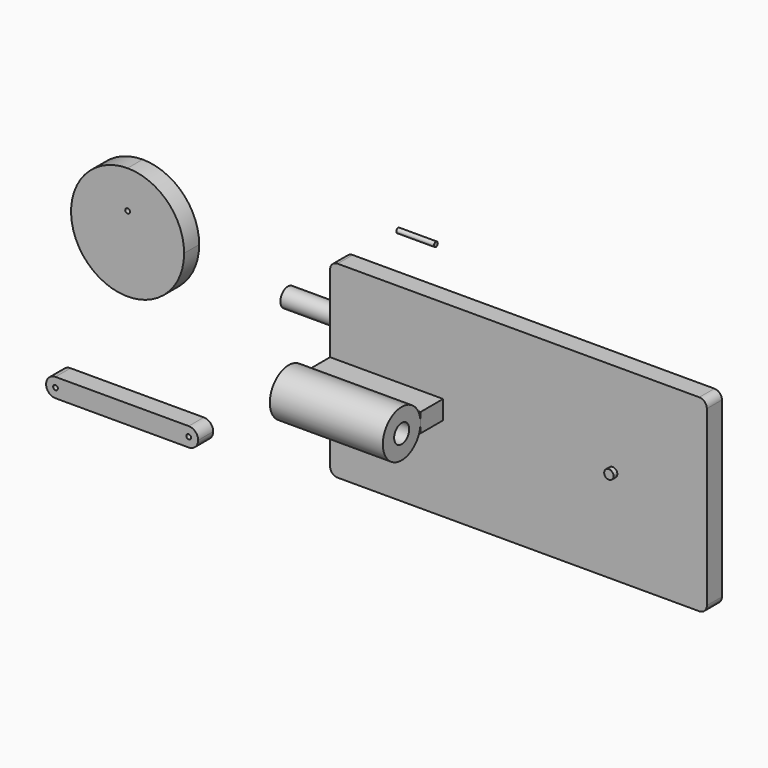
from build123d import *

# Parameters (mm, degrees)
F1_DEPTH  = 254
F0_W      = 19.05
F0_H      = 6.35
F2_DEPTH  = 76.2
F6_DEPTH  = 12.7
F7_R      = 5.08
F9_DEPTH  = 12.7
F10_R     = 6.34999
F11_W     = 52.07
F11_H     = 6.35
F13_DEPTH = 6.35
F14_R     = 6.34999
F15_DEPTH = 3.175
F16_R     = 1.5875
F17_DEPTH = 25.4


# Not quite as in the source:
# - a fillet or chamfer is up to 0.001 mm smaller than in the source, because OpenCascade refuses the exact size


with BuildPart() as f1:
    # F0 (on Right) → F1 (new body)
    with BuildSketch(Plane.YZ):
        Polygon((6.35, -63.5), (6.35, 63.5), (-6.35, 63.5), (-6.35, 6.35), (-6.35, 0), (-6.35, -6.35), (-6.35, -63.5), align=None)
    extrude(amount=F1_DEPTH)

    # F0 (on Right) → F2 (join)
    with BuildSketch(Plane.YZ):
        with Locations((-15.875, 3.175)):
            Rectangle(F0_W, F0_H)
        with Locations((-15.875, -3.175)):
            Rectangle(F0_W, F0_H)
    extrude(amount=F2_DEPTH)

    # F0 (on Right) → F2, piece 2 (join)
    with BuildSketch(Plane.YZ):
        with BuildLine():
            ThreePointArc((-57.15, 0), (-41.275, -15.875), (-25.4, 0))
            Line((-25.4, 0), (-34.925, 0))
            ThreePointArc((-34.925, 0), (-41.275, -6.35), (-47.625, 0))
            Line((-47.625, 0), (-57.15, 0))
        make_face()
        with BuildLine():
            Line((-34.925, 0), (-25.4, 0))
            ThreePointArc((-25.4, 0), (-41.275, 15.875), (-57.15, 0))
            Line((-57.15, 0), (-47.625, 0))
            ThreePointArc((-47.625, 0), (-41.275, 6.35), (-34.925, 0))
        make_face()
    extrude(amount=F2_DEPTH)

    # F7
    f7_edges = [f1.edges().sort_by_distance(p)[0] for p in [
        (254, 0, 63.5),
        (254, 0, -63.5),
        (0, 0, -63.5),
        (0, 0, 63.5),
    ]]
    fillet(f7_edges, radius=F7_R)

    # F5 (on offset) → F15 (join)
    with BuildSketch(Plane.XZ.offset(6.35)):
        with BuildLine():
            Line((190.5, 3.175), (190.5, 0))
            Line((190.5, 0), (193.675, 0))
            ThreePointArc((193.675, 0), (192.745064, 2.245064), (190.5, 3.175))
        make_face()
        with BuildLine():
            Line((187.325, 0), (190.5, 0))
            Line((190.5, 0), (190.5, 3.175))
            ThreePointArc((190.5, 3.175), (188.254936, 2.245064), (187.325, 0))
        make_face()
        with BuildLine():
            Line((190.5, -3.175), (190.5, 0))
            Line((190.5, 0), (187.325, 0))
            ThreePointArc((187.325, 0), (188.254936, -2.245064), (190.5, -3.175))
        make_face()
        with BuildLine():
            Line((193.675, 0), (190.5, 0))
            Line((190.5, 0), (190.5, -3.175))
            ThreePointArc((190.5, -3.175), (192.745064, -2.245064), (193.675, 0))
        make_face()
    extrude(amount=F15_DEPTH)


with BuildPart() as f6:
    # F3 (on Front) → F6 (new body)
    with BuildSketch(Plane.XZ):
        with BuildLine():
            ThreePointArc((-131.435961, 78.357648), (-158.376729, 13.316879), (-93.335961, 40.257648))
            ThreePointArc((-93.335961, 40.257648), (-104.495192, 67.198416), (-131.435961, 78.357648))
        make_face()
        with BuildLine():
            ThreePointArc((-128.260961, 40.257648), (-133.681025, 38.012584), (-131.435961, 43.432648))
            ThreePointArc((-131.435961, 43.432648), (-129.190897, 42.502712), (-128.260961, 40.257648))
        make_face(mode=Mode.SUBTRACT)
        with BuildLine():
            ThreePointArc((-131.435961, 51.370148), (-133.023461, 52.957648), (-131.435961, 54.545148))
            ThreePointArc((-131.435961, 54.545148), (-130.313429, 54.08018), (-129.848461, 52.957648))
            ThreePointArc((-129.848461, 52.957648), (-130.313429, 51.835116), (-131.435961, 51.370148))
        make_face(mode=Mode.SUBTRACT)
        with BuildLine():
            ThreePointArc((-128.260961, 40.257648), (-129.190897, 42.502712), (-131.435961, 43.432648))
            ThreePointArc((-131.435961, 43.432648), (-133.681025, 38.012584), (-128.260961, 40.257648))
        make_face()
    extrude(amount=F6_DEPTH)


with BuildPart() as f9:
    # F8 (on Front) → F9 (new body)
    with BuildSketch(Plane.XZ):
        with BuildLine():
            Line((-186.38583, -67.65892), (-186.38583, -74.00892))
            Line((-186.38583, -74.00892), (-180.03583, -74.00892))
            Line((-180.03583, -74.00892), (-180.03583, -69.24642))
            ThreePointArc((-180.03583, -69.24642), (-181.158362, -68.781452), (-181.62333, -67.65892))
            Line((-181.62333, -67.65892), (-186.38583, -67.65892))
        make_face()
        with BuildLine():
            Line((-180.03583, -69.24642), (-180.03583, -74.00892))
            Line((-180.03583, -74.00892), (-135.13455, -74.00892))
            Line((-135.13455, -74.00892), (-135.13455, -61.30892))
            Line((-135.13455, -61.30892), (-180.03583, -61.30892))
            Line((-180.03583, -61.30892), (-180.03583, -66.07142))
            ThreePointArc((-180.03583, -66.07142), (-178.913298, -66.536388), (-178.44833, -67.65892))
            ThreePointArc((-178.44833, -67.65892), (-178.913298, -68.781452), (-180.03583, -69.24642))
        make_face()
        with BuildLine():
            Line((-186.38583, -61.30892), (-186.38583, -67.65892))
            Line((-186.38583, -67.65892), (-181.62333, -67.65892))
            ThreePointArc((-181.62333, -67.65892), (-181.158362, -66.536388), (-180.03583, -66.07142))
            Line((-180.03583, -66.07142), (-180.03583, -61.30892))
            Line((-180.03583, -61.30892), (-186.38583, -61.30892))
        make_face()
        with BuildLine():
            Line((-135.13455, -61.30892), (-135.13455, -74.00892))
            Line((-135.13455, -74.00892), (-90.233269, -74.00892))
            Line((-90.233269, -74.00892), (-90.233269, -69.24642))
            ThreePointArc((-90.233269, -69.24642), (-91.820769, -67.65892), (-90.233269, -66.07142))
            Line((-90.233269, -66.07142), (-90.233269, -61.30892))
            Line((-90.233269, -61.30892), (-135.13455, -61.30892))
        make_face()
        with BuildLine():
            Line((-90.233269, -69.24642), (-90.233269, -74.00892))
            Line((-90.233269, -74.00892), (-83.883269, -74.00892))
            Line((-83.883269, -74.00892), (-83.883269, -67.65892))
            Line((-83.883269, -67.65892), (-88.645769, -67.65892))
            ThreePointArc((-88.645769, -67.65892), (-89.110737, -68.781452), (-90.233269, -69.24642))
        make_face()
        with BuildLine():
            Line((-83.883269, -61.30892), (-90.233269, -61.30892))
            Line((-90.233269, -61.30892), (-90.233269, -66.07142))
            ThreePointArc((-90.233269, -66.07142), (-89.110737, -66.536388), (-88.645769, -67.65892))
            Line((-88.645769, -67.65892), (-83.883269, -67.65892))
            Line((-83.883269, -67.65892), (-83.883269, -61.30892))
        make_face()
    extrude(amount=F9_DEPTH)

    # F10 (radius 6.35 in the source; OpenCascade refuses exactly that, so slightly less here)
    f10_edges = [f9.edges().sort_by_distance(p)[0] for p in [
        (-83.883269, -6.35, -61.30892),
        (-83.883269, -6.35, -74.00892),
        (-186.38583, -6.35, -61.30892),
        (-186.38583, -6.35, -74.00892),
    ]]
    fillet(f10_edges, radius=F10_R)


with BuildPart() as f12:
    # F11 (on Top) → F12 (revolve)
    with BuildSketch(Plane.XY):
        with Locations((-41.717986, 45.964235)):
            Rectangle(F11_W, F11_H)
    revolve(axis=Axis((-32.827986, 42.789235, 0), (1, 0, 0)))

    # F11 (on Top) → F13 (join, symmetric)
    with BuildSketch(Plane.XY):
        with BuildLine():
            Line((-15.682986, 49.139235), (-15.682986, 42.789235))
            Line((-15.682986, 42.789235), (-5.840486, 42.789235))
            ThreePointArc((-5.840486, 42.789235), (-5.375518, 43.911767), (-4.252986, 44.376735))
            Line((-4.252986, 44.376735), (-4.252986, 49.139235))
            Line((-4.252986, 49.139235), (-15.682986, 49.139235))
        make_face()
        with BuildLine():
            Line((-4.252986, 49.139235), (-4.252986, 44.376735))
            ThreePointArc((-4.252986, 44.376735), (-3.130454, 43.911767), (-2.665486, 42.789235))
            Line((-2.665486, 42.789235), (2.097014, 42.789235))
            Line((2.097014, 42.789235), (2.097014, 49.139235))
            Line((2.097014, 49.139235), (-4.252986, 49.139235))
        make_face()
        with BuildLine():
            ThreePointArc((-2.665486, 42.789235), (-3.130454, 41.666703), (-4.252986, 41.201735))
            Line((-4.252986, 41.201735), (-4.252986, 36.439235))
            Line((-4.252986, 36.439235), (2.097014, 36.439235))
            Line((2.097014, 36.439235), (2.097014, 42.789235))
            Line((2.097014, 42.789235), (-2.665486, 42.789235))
        make_face()
        with BuildLine():
            Line((-5.840486, 42.789235), (-15.682986, 42.789235))
            Line((-15.682986, 42.789235), (-15.682986, 36.439235))
            Line((-15.682986, 36.439235), (-4.252986, 36.439235))
            Line((-4.252986, 36.439235), (-4.252986, 41.201735))
            ThreePointArc((-4.252986, 41.201735), (-5.375518, 41.666703), (-5.840486, 42.789235))
        make_face()
    extrude(amount=F13_DEPTH, both=True)

    # F14 (radius 6.35 in the source; OpenCascade refuses exactly that, so slightly less here)
    f14_edges = [f12.edges().sort_by_distance(p)[0] for p in [
        (2.097014, 49.139235, 0),
        (2.097014, 36.439235, 0),
    ]]
    fillet(f14_edges, radius=F14_R)


with BuildPart() as f17:
    # F16 (on Right) → F17 (new body)
    with BuildSketch(Plane.YZ):
        with Locations((51.06695, 58.249027)):
            Circle(F16_R)
    extrude(amount=F17_DEPTH)


solid = Compound([f1.part, f6.part, f9.part, f12.part, f17.part])
